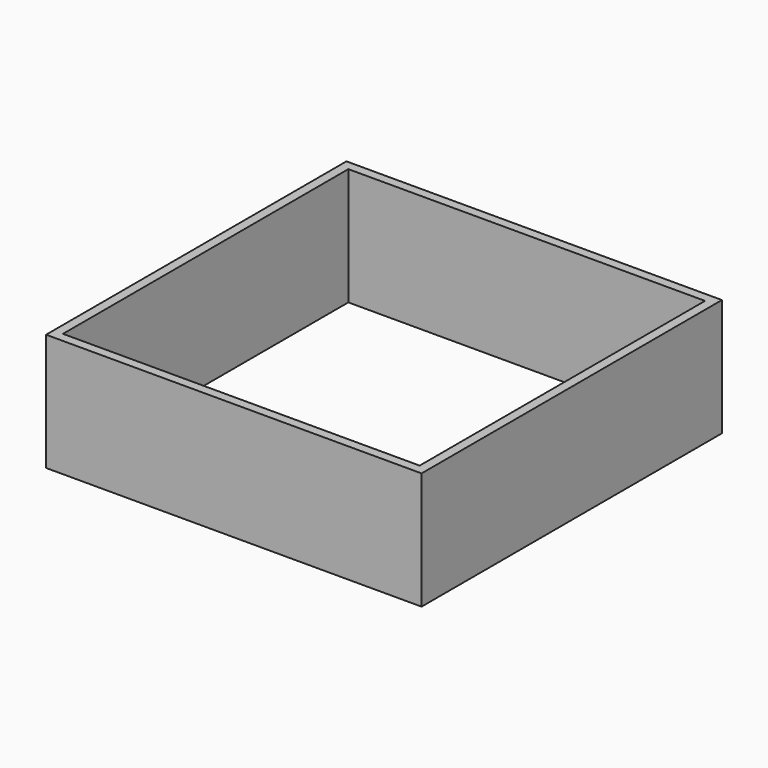
from build123d import *

# Parameters (mm, degrees)
F0_W     = 80
F0_H     = 80
F0_W_2   = 76
F0_H_2   = 76
F1_DEPTH = 25
F2_W     = 12.4
F2_H     = 10
F3_DEPTH = 11.5
F4_R     = 4.99999
F5_R     = 1.9
F6_DEPTH = 25
F7_W     = 6.50001
F7_H     = 4.2
F7_W_2   = 4.99999
F8_DEPTH = 25


# Not quite as in the source:
# - a fillet or chamfer is up to 0.001 mm smaller than in the source, because OpenCascade refuses the exact size


with BuildPart() as f1:
    # F0 (on Top) → F1 (new body)
    with BuildSketch(Plane.XY):
        Rectangle(F0_W, F0_H)
        Rectangle(F0_W_2, F0_H_2, mode=Mode.SUBTRACT)
    extrude(amount=F1_DEPTH)

    # F2 (on face) → F3 (join)
    with BuildSketch(Plane(origin=(-40, 0, 0), x_dir=(0, -1, 0), z_dir=(-1, 0, 0))):
        with Locations((0, 5)):
            Rectangle(F2_W, F2_H)
    extrude(amount=F3_DEPTH)

    # F4 (radius 5 in the source; OpenCascade refuses exactly that, so slightly less here)
    f4_edges = [f1.edges().sort_by_distance(p)[0] for p in [
        (-51.5, 0, 10),
        (-51.5, 0, 0),
    ]]
    fillet(f4_edges, radius=F4_R)

    # F5 (on face) → F6 (cut)
    with BuildSketch(Plane(origin=(0, 6.2, 0), x_dir=(-1, 0, 0), z_dir=(0, 1, 0))):
        with Locations((46.5, 5)):
            Circle(F5_R)
    extrude(amount=-F6_DEPTH, mode=Mode.SUBTRACT)

    # F7 (on face) → F8 (cut)
    with BuildSketch(Plane.XY.offset(10)):
        with Locations((-43.250005, 0)):
            Rectangle(F7_W, F7_H)
        with Locations((-49.000005, 0)):
            Rectangle(F7_W_2, F7_H)
    extrude(amount=-F8_DEPTH, mode=Mode.SUBTRACT)


solid = f1.part
